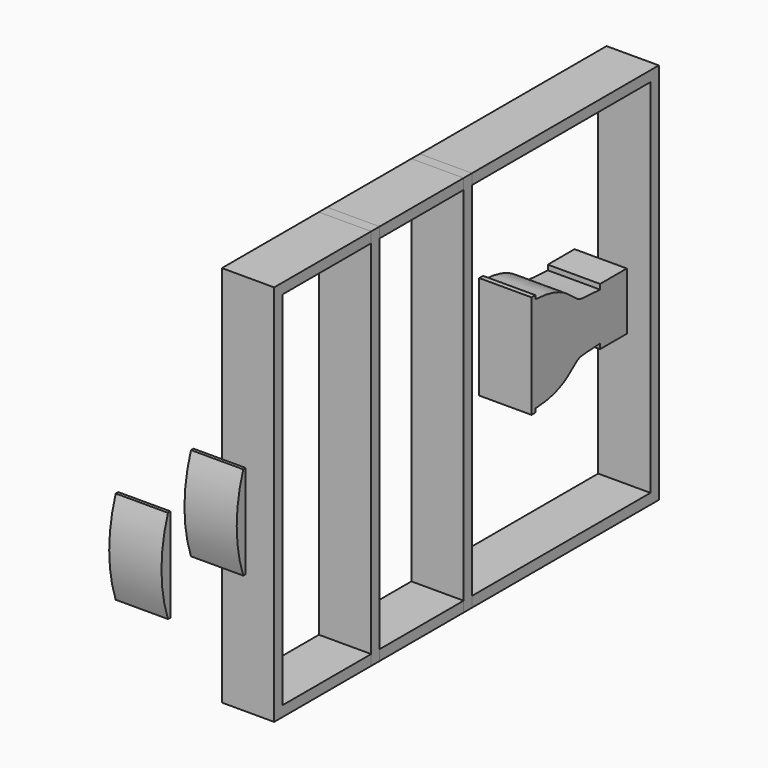
from build123d import *

# Parameters (mm, degrees)
F3_W     = 230
F3_H     = 183
F3_W_2   = 220
F3_H_2   = 173
F4_DEPTH = 25
F5_DEPTH = 25
F6_W     = 5
F6_H     = 183
F7_DEPTH = 25


# Not quite as in the source:
# - the dataset's text gives a spline's control points without its knots; the knots are read off the source's solid


with BuildPart() as f4:
    # F3 (on Right) → F4 (new body)
    with BuildSketch(Plane.YZ):
        with Locations((115, 0)):
            Rectangle(F3_W, F3_H)
        with Locations((115, 0)):
            Rectangle(F3_W_2, F3_H_2, mode=Mode.SUBTRACT)
    extrude(amount=F4_DEPTH)


with BuildPart() as f5:
    # F2 (on Right) → F5 (new body)
    with BuildSketch(Plane.YZ):
        with BuildLine():
            Line((210.8721694193, -13.75), (210.8721694193, 13.75))
            Line((210.8721694193, 13.75), (194.8721694193, 13.75))
            Line((194.8721694193, 13.75), (194.8721694193, 11.3520892337))
            add(Edge.make_bspline(
                [(156.1721694193, 22.9873415195), (172.6975398433, 22.3892458961), (180.3810074103, 10.6525710072), (185.9791283701, 12.0223834249), (194.8721694193, 11.3520892337)],
                knots=[0, 0, 0, 0, 0.5786049699, 1, 1, 1, 1], degree=3))
            Line((156.1721694193, 22.9873415195), (156.1721694193, 24.75))
            Line((156.1721694193, 24.75), (153.8721694193, 24.75))
            Line((153.8721694193, 24.75), (153.8721694193, -24.75))
            Line((153.8721694193, -24.75), (156.1721694193, -24.75))
            Line((156.1721694193, -24.75), (156.1721694193, -22.9873415195))
            add(Edge.make_bspline(
                [(156.1721694193, -22.9873415195), (172.6975398433, -22.3892458961), (180.3810074103, -10.6525710072), (185.9791283701, -12.0223834249), (194.8721694193, -11.3520892337)],
                knots=[0, 0, 0, 0, 0.5786049699, 1, 1, 1, 1], degree=3))
            Line((194.8721694193, -11.3520892337), (194.8721694193, -13.75))
            Line((194.8721694193, -13.75), (210.8721694193, -13.75))
        make_face()
    extrude(amount=F5_DEPTH)


with BuildPart() as f5b:
    # F2 (on Right) → F5, piece 2 (new body)
    with BuildSketch(Plane.YZ):
        with BuildLine():
            Line((-17, 22.375), (-18.5, 22.375))
            ThreePointArc((-18.5, 22.375), (-22.4, 0), (-18.5, -22.375))
            Line((-18.5, -22.375), (-17, -22.375))
            Line((-17, -22.375), (-17, 22.375))
        make_face()
    extrude(amount=F5_DEPTH)


with BuildPart() as f5c:
    # F2 (on Right) → F5, piece 3 (new body)
    with BuildSketch(Plane.YZ):
        with BuildLine():
            Line((-62, 22.375), (-63.5, 22.375))
            ThreePointArc((-63.5, 22.375), (-67.4, 0), (-63.5, -22.375))
            Line((-63.5, -22.375), (-62, -22.375))
            Line((-62, -22.375), (-62, 22.375))
        make_face()
    extrude(amount=F5_DEPTH)


with BuildPart() as f7:
    # F6 (on Right) → F7 (new body)
    with BuildSketch(Plane.YZ):
        with Locations((60.5, 0)):
            Rectangle(F6_W, F6_H)
    extrude(amount=F7_DEPTH)


with BuildPart() as f7b:
    # F6 (on Right) → F7, piece 2 (new body)
    with BuildSketch(Plane.YZ):
        with Locations((115.8, 0)):
            Rectangle(F6_W, F6_H)
    extrude(amount=F7_DEPTH)


solid = Compound([f4.part, f5.part, f5b.part, f5c.part, f7.part, f7b.part])
